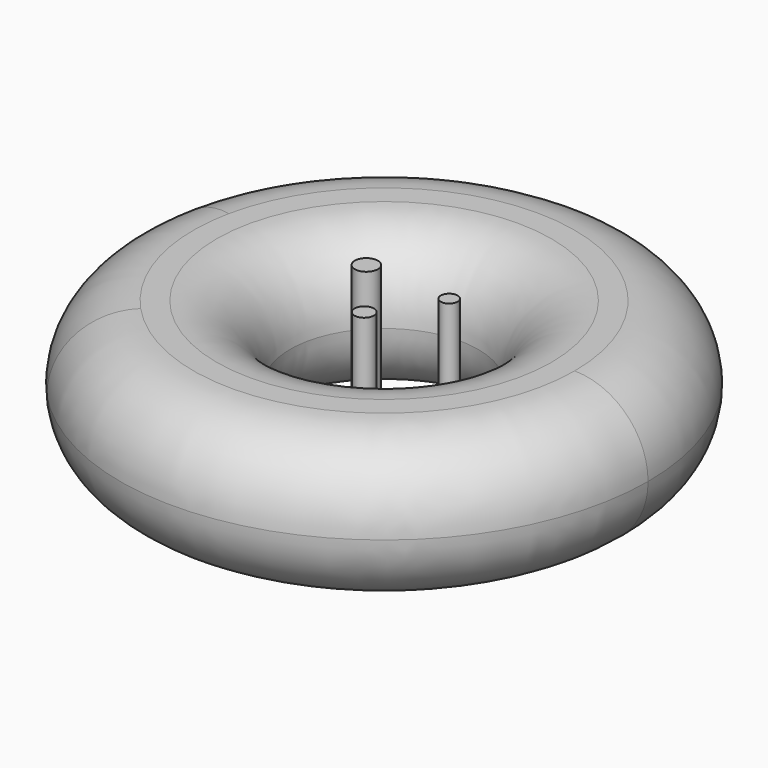
from build123d import *

# Parameters (mm, degrees)
F0_R     = 16.2559412927
F1_DEPTH = 25.4
F0_R_2   = 1.6786130333
F0_R_3   = 2.0024582602
F0_R_4   = 1.4602850905
F2_R     = 12.69999


# Not quite as in the source:
# - a fillet or chamfer is up to 0.001 mm smaller than in the source, because OpenCascade refuses the exact size


with BuildPart() as f1:
    # F0 (on Top) → F1 (new body)
    with BuildSketch(Plane.XY):
        with BuildLine():
            ThreePointArc((-33.5562936962, -30.9732549017), (16.6281629524, -42.5308307309), (45.6658227324, 0))
            ThreePointArc((45.6658227324, 0), (4.7136039757, 45.421903344), (-44.6927509203, 9.3768534705))
            ThreePointArc((-44.6927509203, 9.3768534705), (-44.0200074655, -12.1493336678), (-33.5562936962, -30.9732549017))
        make_face()
        Circle(F0_R, mode=Mode.SUBTRACT)
    extrude(amount=F1_DEPTH)

    # F2 (radius 12.7 in the source; OpenCascade refuses exactly that, so slightly less here)
    f2_edges = [f1.edges().sort_by_distance(p)[0] for p in [
        (-45.665823, 0, 0),
        (45.665823, 0, 12.7),
        (-45.665823, 0, 25.4),
        (16.255941, 0, 12.7),
        (-16.255941, 0, 0),
        (-16.255941, 0, 25.4),
    ]]
    fillet(f2_edges, radius=F2_R)


with BuildPart() as f1b:
    # F0 (on Top) → F1, piece 2 (new body)
    with BuildSketch(Plane.XY):
        with Locations((0, -4.3064509518)):
            Circle(F0_R_2)
    extrude(amount=F1_DEPTH)


with BuildPart() as f1c:
    # F0 (on Top) → F1, piece 3 (new body)
    with BuildSketch(Plane.XY):
        with Locations((-8.3801168948, 6.6342614591)):
            Circle(F0_R_3)
    extrude(amount=F1_DEPTH)


with BuildPart() as f1d:
    # F0 (on Top) → F1, piece 4 (new body)
    with BuildSketch(Plane.XY):
        with Locations((6.5178754739, 5.9359185398)):
            Circle(F0_R_4)
    extrude(amount=F1_DEPTH)


solid = Compound([f1.part, f1b.part, f1c.part, f1d.part])
